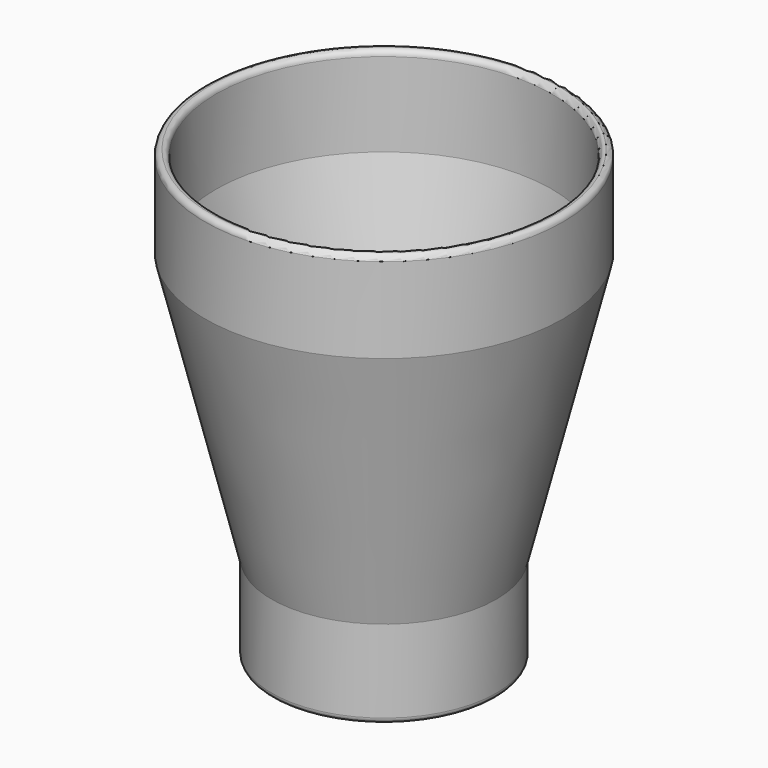
from build123d import *

# Parameters (mm, degrees)
F3_DEPTH = 25.4
F5_DEPTH = 25.4
F6_R     = 1.58749


# Not quite as in the source:
# - a fillet or chamfer is up to 0.001 mm smaller than in the source, because OpenCascade refuses the exact size


with BuildPart() as f1:
    # F0 (on Front) → F1 (revolve)
    with BuildSketch(Plane.XZ):
        Polygon((28.702, 25.4), (28.702, 0), (31.877, 0), (31.877, 25.0116683196), (50.8, 101.2116683196), (50.8, 127), (47.625, 127), (47.625, 101.6), align=None)
    revolve(axis=Axis((0, 0, 50.8), (0, 0, 1)))

    # F2 (on Right) → F3 (cut)
    with BuildSketch(Plane.YZ):
        with BuildLine():
            Line((0, 0), (9.525, 0))
            Line((9.525, 0), (9.525, 10.033))
            ThreePointArc((9.525, 10.033), (8.5950640303, 12.2780640303), (6.35, 13.208))
            Line((6.35, 13.208), (-2.778125, 13.208))
            Line((-2.778125, 13.208), (-3.6299686429, 12.7091803589))
            ThreePointArc((-3.6299686429, 12.7091803589), (-9.5245978264, 9.1827514033), (-3.5319644808, 5.825565085))
            Line((-3.5319644808, 5.825565085), (-2.778125, 5.2705))
            Line((-2.778125, 5.2705), (0, 5.2705))
            Line((0, 5.2705), (0, 0))
        make_face()
    extrude(amount=-F3_DEPTH, mode=Mode.SUBTRACT)

    # F4 (on Right) → F5 (cut)
    with BuildSketch(Plane.YZ):
        with BuildLine():
            Line((-9.5220467116, 9.9028743273), (-9.5220467116, -0.1301256727))
            Line((-9.5220467116, -0.1301256727), (0.0029532884, -0.1301256727))
            Line((0.0029532884, -0.1301256727), (0.0029532884, 5.1403743273))
            Line((0.0029532884, 5.1403743273), (2.7810782884, 5.1403743273))
            Line((2.7810782884, 5.1403743273), (3.5349177692, 5.6954394123))
            ThreePointArc((3.5349177692, 5.6954394123), (9.5275511148, 9.0526257306), (3.6329219313, 12.5790546862))
            Line((3.6329219313, 12.5790546862), (2.7810782884, 13.0778743273))
            Line((2.7810782884, 13.0778743273), (-6.3470467116, 13.0778743273))
            ThreePointArc((-6.3470467116, 13.0778743273), (-8.5921107418, 12.1479383576), (-9.5220467116, 9.9028743273))
        make_face()
    extrude(amount=F5_DEPTH, mode=Mode.SUBTRACT)

    # F6 (radius 1.5875 in the source; OpenCascade refuses exactly that, so slightly less here)
    f6_edges = [f1.edges().sort_by_distance(p)[0] for p in [
        (-31.877, 0, 0),
        (-50.8, 0, 127),
        (-28.702, 0, 0),
        (-47.625, 0, 127),
    ]]
    fillet(f6_edges, radius=F6_R)


solid = f1.part
